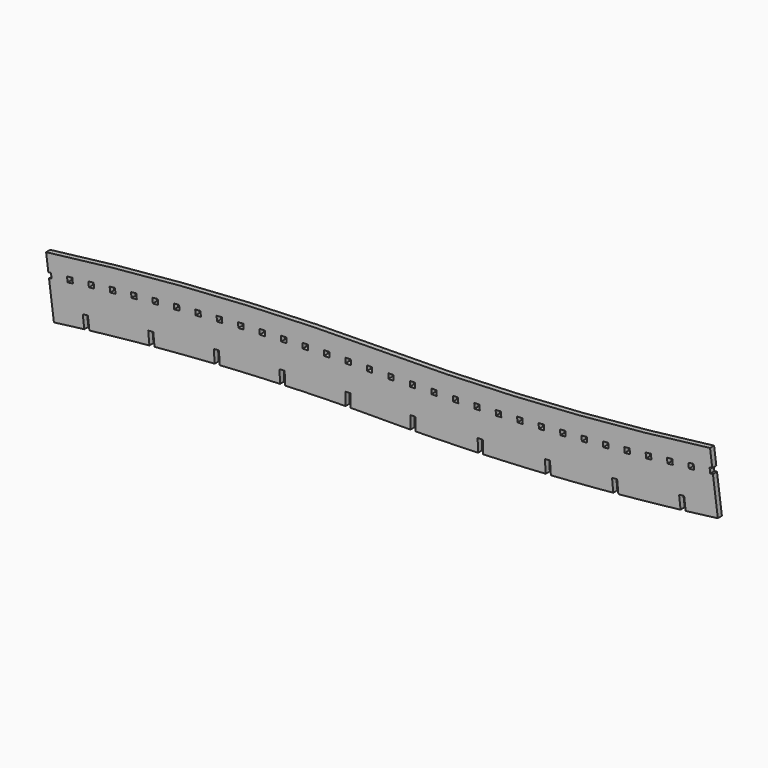
from build123d import *

# Parameters (mm, degrees)
F1_W             = 3
F1_H             = 35
F5_DEPTH         = 406
F5_COPIES_COUNT  = 16
F5_COPIES_ANGLE  = 7.2580645161
F7_DEPTH         = 3
F7_COPIES_COUNT  = 16
F7_COPIES_ANGLE  = 7.2580645161
F9_DEPTH         = 3
F9_COPIES_COUNT  = 5
F9_COPIES_ANGLE  = 6
F11_DEPTH        = 3
F11_COPIES_COUNT = 5
F11_COPIES_ANGLE = 6


# Not quite as in the source:
# - an extrude ends at something that could not be found from the text; its depth is read off the source's solid
# - a pattern or mirror of a feature is missing from the dataset's text; its kind, count and spacing are read off the source's solid


with BuildPart() as f2:
    # F2: sweep along a path in F0
    with BuildLine(Plane.XZ) as f2_path:
        ThreePointArc((-194.2229740234, -12.7300462758), (-97.3198562945, -3.185922221), (0, 0))
    # F1 (on Right) → F2 (sweep)
    with BuildSketch(Plane.YZ):
        with Locations((-1.5, -7.5)):
            Rectangle(F1_W, F1_H)
    sweep(path=f2_path.line)

    # F3: sweep along a path in F0
    with BuildLine(Plane.XZ) as f3_path:
        ThreePointArc((0, 0), (97.3198562945, 3.185922221), (194.2229740234, 12.7300462758))
    # F1 (on Right) → F3 (sweep)
    with BuildSketch(Plane.YZ):
        with Locations((-1.5, -7.5)):
            Rectangle(F1_W, F1_H)
    sweep(path=f3_path.line)

    # F4 (on Front) → F5 (cut, through all)
    with BuildSketch(Plane.XZ):
        Polygon((195.7803319699, 12.9350763391), (194.2229740234, 12.7300462758), (194.6145526001, 9.7557116916), (196.1719105466, 9.9607417549), align=None)
        Polygon((194.6145526001, 9.7557116916), (194.2229740234, 12.7300462758), (192.665616077, 12.5250162125), (193.0571946536, 9.5506816284), align=None)
    f5 = extrude(amount=F5_DEPTH, mode=Mode.SUBTRACT)

    # F5_copies: F5 ×16 about axis
    f5_copies_axis = Axis((0, 0, 1488), (0, 1, 0))
    for i in range(1, F5_COPIES_COUNT):
        add(f5.rotate(f5_copies_axis, i * F5_COPIES_ANGLE / (F5_COPIES_COUNT - 1)), mode=Mode.SUBTRACT)

    # F6 (on face) → F7 (cut, through all)
    with BuildSketch(Plane.XZ.offset(3)):
        Polygon((-192.665616077, -12.5250162125), (-195.7803319699, -12.9350763391), (-195.3887533932, -15.9094109232), (-192.2740375003, -15.4993507966), align=None)
    f7 = extrude(amount=-F7_DEPTH, mode=Mode.SUBTRACT)

    # F7_copies: F7 ×16 about axis
    f7_copies_axis = Axis((0, 0, -1488), (0, 1, 0))
    for i in range(1, F7_COPIES_COUNT):
        add(f7.rotate(f7_copies_axis, i * F7_COPIES_ANGLE / (F7_COPIES_COUNT - 1)), mode=Mode.SUBTRACT)

    # F8 (on face) → F9 (cut, through all)
    with BuildSketch(Plane.XZ.offset(3)):
        Polygon((-171.0720633571, -27.4848211661), (-174.051335548, -27.8368683399), (-173.1712176135, -35.2850488171), (-170.1919454226, -34.9330016433), align=None)
    f9 = extrude(amount=-F9_DEPTH, mode=Mode.SUBTRACT)

    # F9_copies: F9 ×5 about axis
    f9_copies_axis = Axis((0, 0, -1488), (0, 1, 0))
    for i in range(1, F9_COPIES_COUNT):
        add(f9.rotate(f9_copies_axis, i * F9_COPIES_ANGLE / (F9_COPIES_COUNT - 1)), mode=Mode.SUBTRACT)

    # F10 (on face) → F11 (cut, through all)
    with BuildSketch(Plane.XZ.offset(3)):
        Polygon((174.8095745253, -7.316646917), (175.7464026416, -15.2616046313), (178.7257617845, -14.9102940876), (177.7889336681, -6.9653363734), align=None)
    f11 = extrude(amount=-F11_DEPTH, mode=Mode.SUBTRACT)

    # F11_copies: F11 ×5 about axis
    f11_copies_axis = Axis((0, 0, 1488), (0, 1, 0))
    for i in range(1, F11_COPIES_COUNT):
        add(f11.rotate(f11_copies_axis, i * F11_COPIES_ANGLE / (F11_COPIES_COUNT - 1)), mode=Mode.SUBTRACT)


solid = f2.part
